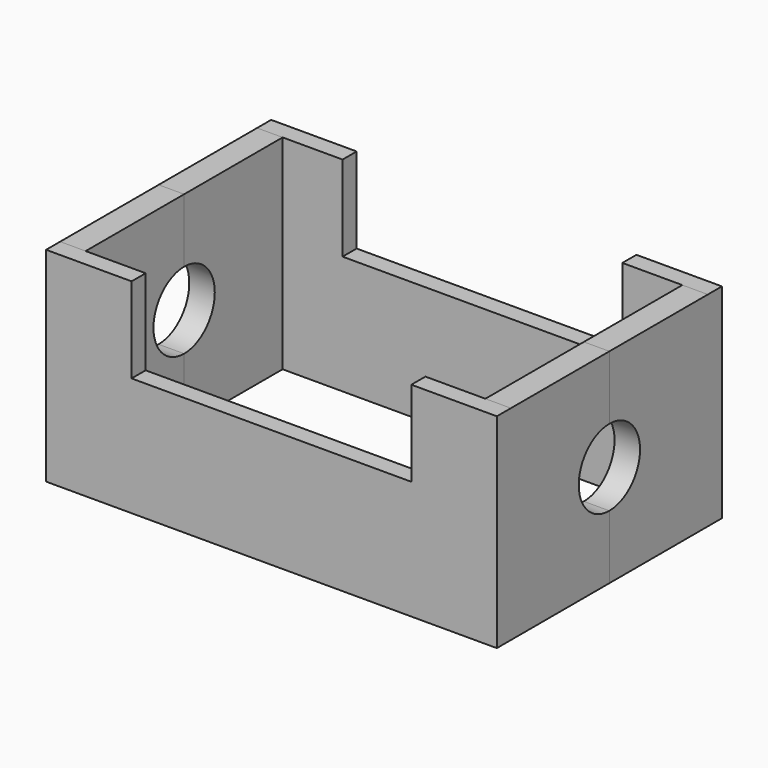
from build123d import *
from build123d import SkipClean  # not in build123d's __all__

# Parameters (mm, degrees)
F0_W     = 4.6070814133
F0_H     = 36.8574000895
F1_DEPTH = 3.175
F2_DEPTH = 25.4
F4_DEPTH = 6.35


# Not quite as in the source:
# - a feature names something its author has since deleted; it is built from what else it names


with BuildPart() as f1:
    # F0 (on Front) → F1 (new body)
    with BuildSketch(Plane.XZ):
        with Locations((38.3936055005, 18.4287000448)):
            Rectangle(F0_W, F0_H)
        Polygon((0, 21.4239992201), (0, 0), (36.0900647938, 0), (36.0900647938, 36.8574000895), (25.2613946795, 36.8574000895), (25.2613946795, 21.4239992201), align=None)
        Polygon((0, 21.4239992201), (0, 0), (36.0900647938, 0), (36.0900647938, 36.8574000895), (25.2613946795, 36.8574000895), (25.2613946795, 21.4239992201), align=None)
    extrude(amount=F1_DEPTH)

    # F0 (on Front) → F2 (join)
    with BuildSketch(Plane.XZ):
        with Locations((38.3936055005, 18.4287000448)):
            Rectangle(F0_W, F0_H)
    extrude(amount=F2_DEPTH)

    # F3 (on face) → F4 (cut)
    with BuildSketch(Plane.YZ.offset(40.6971462071)):
        with BuildLine():
            Line((-25.4, 25.344834663), (-25.4, 11.5125654265))
            ThreePointArc((-25.4, 11.5125654265), (-18.4838653818, 18.4287000448), (-25.4, 25.344834663))
        make_face()
    extrude(amount=-F4_DEPTH, mode=Mode.SUBTRACT)

    # F5: F1 across plane


with BuildPart() as f1_1:
    add(f1.part, clean=False)
    add(f1.part.mirror(Plane.YZ), clean=False)

    # F6: F1 across face


with BuildPart() as f1_2:
    add(f1_1.part, clean=False)
    with SkipClean():  # cleaning this boolean's faces spoils the solid; the shape is the same uncleaned
        add(f1_1.part.mirror(Plane(origin=(38.3936055005, -25.4, 5.7562827133), x_dir=(1, 0, 0), z_dir=(0, -1, 0))), clean=False)


solid = f1_2.part
